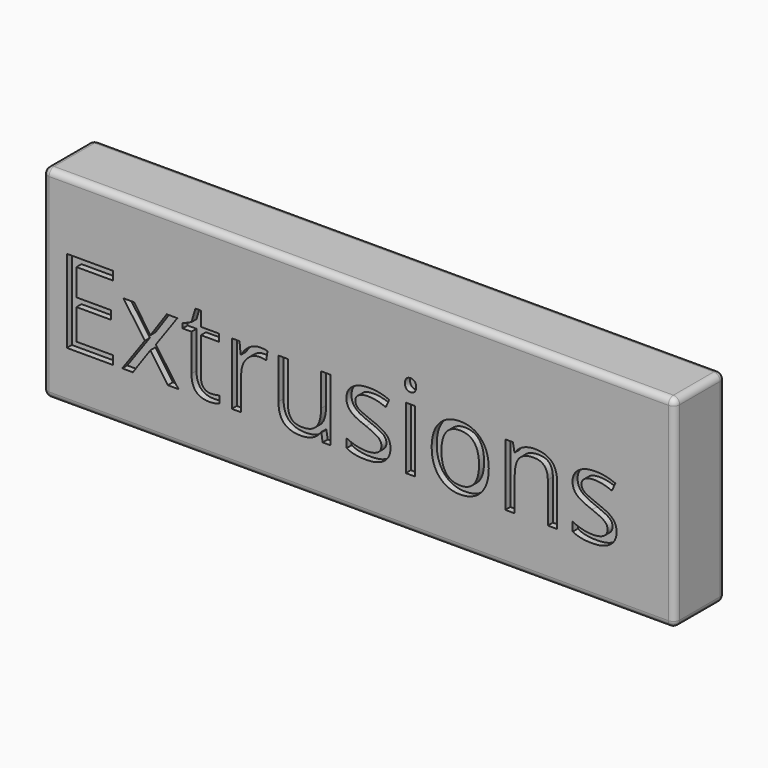
from build123d import *

# Parameters (mm, degrees)
F0_W         = 500
F0_H         = 50
F1_DEPTH     = 160
F2_R         = 5
F3_TEXT_SIZE = 91.8601684103
F4_DEPTH     = 5


# Not quite as in the source:
# - Text() gives the source's letters only with a copy of the font that has no kerning and outlines rounded to 1/6400 em; it was checked with that copy


with BuildPart() as f1:
    # F0 (on Top) → F1 (new body)
    with BuildSketch(Plane.XY):
        with Locations((-250, -25)):
            Rectangle(F0_W, F0_H)
    extrude(amount=F1_DEPTH)

    # F2
    f2_edges = [f1.edges().sort_by_distance(p)[0] for p in [
        (0, -50, 80),
        (0, 0, 80),
        (0, -25, 160),
        (-250, 0, 160),
        (-500, -25, 160),
        (-250, -50, 160),
        (-500, -50, 80),
        (-250, -50, 0),
        (-500, 0, 80),
        (-500, -25, 0),
        (-250, 0, 0),
        (0, -25, 0),
    ]]
    fillet(f2_edges, radius=F2_R)

    # F3 (on face) → F4 (cut)
    with BuildSketch(Plane.XZ.offset(50)):
        with Locations((-490, 40.1890069986)):
            Text('Extrusions', F3_TEXT_SIZE, font='Open Sans', text_align=(TextAlign.LEFT, TextAlign.BOTTOM))
    extrude(amount=-F4_DEPTH, mode=Mode.SUBTRACT)


solid = f1.part
